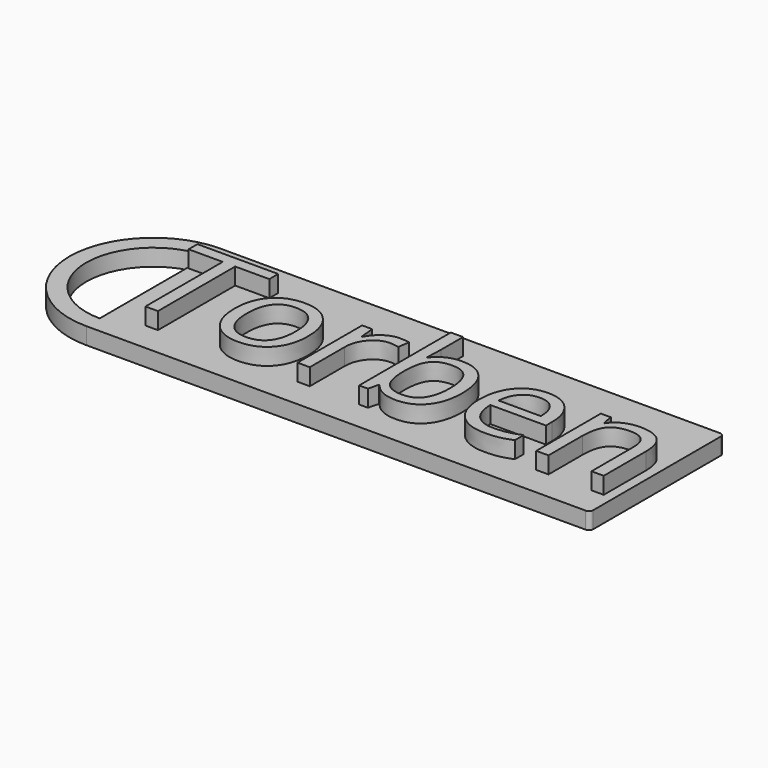
from build123d import *

# Parameters (mm, degrees)
F4_DEPTH     = 2
F1_R         = 0.5
F2_TEXT_SIZE = 17.9766864847
F3_DEPTH     = 2


# Not quite as in the source:
# - Text() gives the source's letters only with a copy of the font that has no kerning and outlines rounded to 1/6400 em; it was checked with that copy


with BuildPart() as f4:
    # F0 (on Top) → F4 (new body)
    with BuildSketch(Plane.XY):
        Polygon((54.7291392038, 3.2207785361), (-5.2708607962, 3.2207785361), (-5.2708607962, 1.2207785361), (-5.2708607962, -14.7792214639), (-5.2708607962, -16.7792214639), (54.7291392038, -16.7792214639), align=None)
        with BuildLine():
            Line((-5.2708607962, 1.2207785361), (-5.2708607962, 3.2207785361))
            ThreePointArc((-5.2708607962, 3.2207785361), (-15.2708607962, -6.7792214639), (-5.2708607962, -16.7792214639))
            Line((-5.2708607962, -16.7792214639), (-5.2708607962, -14.7792214639))
            ThreePointArc((-5.2708607962, -14.7792214639), (-13.2708607962, -6.7792214639), (-5.2708607962, 1.2207785361))
        make_face()
    extrude(amount=F4_DEPTH)

    # F1
    f1_edges = [f4.edges().sort_by_distance(p)[0] for p in [
        (54.729139, -16.779221, 1),
        (54.729139, 3.220779, 1),
    ]]
    fillet(f1_edges, radius=F1_R)

    # F2 (on face) → F3 (join)
    with BuildSketch(Plane.XY.offset(2)):
        with Locations((-5.2708607962, -13.2508285984)):
            Text('Torben', F2_TEXT_SIZE, font='Open Sans', text_align=(TextAlign.LEFT, TextAlign.BOTTOM))
    extrude(amount=F3_DEPTH)


solid = f4.part
